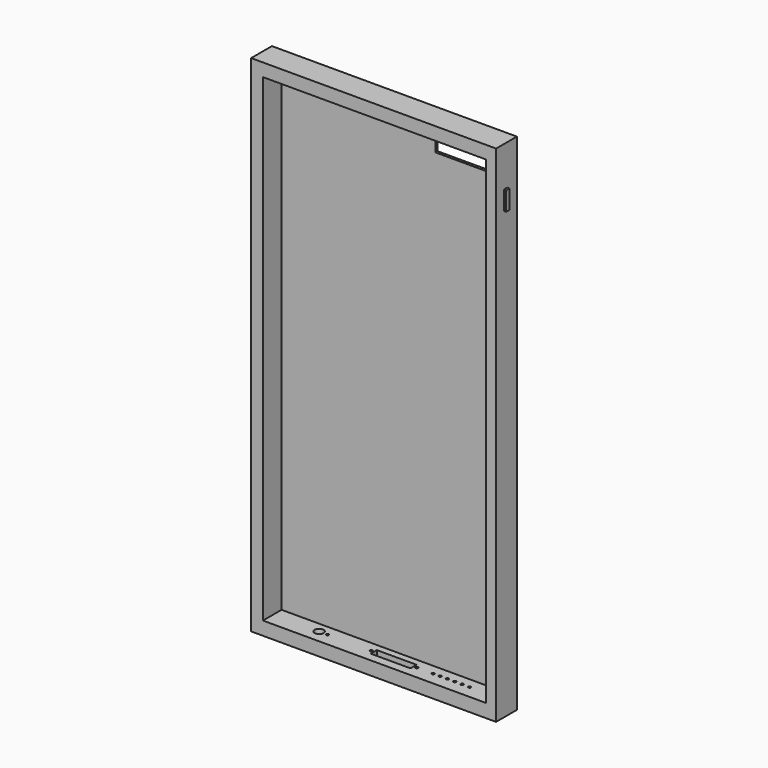
from build123d import *

# Parameters (mm, degrees)
F0_W          = 67.056
F0_H          = 138.176
F1_DEPTH      = 7.112
F2_W          = 1.1457276996
F2_H          = 5.1557719707
F3_DEPTH      = 0.6604
F4_W          = 1.0838428756
F4_H          = 4.3208114803
F5_DEPTH      = 0.7874
F6_W          = 0.8028652519
F6_H          = 3.1311772764
F6_H_2        = 3.1713172793
F7_DEPTH      = 0.4826
F8_W          = 61.0314477235
F8_H          = 130.9745721519
F9_DEPTH      = 6.3754
F10_W         = 17.1431452036
F10_H         = 5.4619573057
F11_DEPTH     = 25.4
F12_TEXT_SIZE = 1.3546895893
F13_DEPTH     = 0.127
F14_TEXT_SIZE = 2.2497099878
F15_DEPTH     = 0.127
F16_R         = 1.2281483903
F17_DEPTH     = 25.4
F18_R         = 0.3683
F19_DEPTH     = 25.4
F20_W         = 10.8844151255
F20_H         = 2.1005012095
F21_DEPTH     = 25.4
F22_DEPTH     = 25.4


# Not quite as in the source:
# - Text() gives the source's letters only with a copy of the font that has no kerning and outlines rounded to 1/6400 em; it was checked with that copy


with BuildPart() as f1:
    # F0 (on Front) → F1 (new body)
    with BuildSketch(Plane.XZ):
        with Locations((-11.8578484981, -4.7733456488)):
            Rectangle(F0_W, F0_H)
    extrude(amount=F1_DEPTH)

    # F2 (on face) → F3 (join)
    with BuildSketch(Plane.YZ.offset(21.6701515019)):
        with Locations((-3.914569621, 50.7939383388)):
            Rectangle(F2_W, F2_H)
    extrude(amount=F3_DEPTH)

    # F4 (on face) → F5 (cut)
    with BuildSketch(Plane(origin=(-45.3858484981, 0, 0), x_dir=(0, -1, 0), z_dir=(-1, 0, 0))):
        with Locations((3.0140785622, 55.3201716393)):
            Rectangle(F4_W, F4_H)
    extrude(amount=-F5_DEPTH, mode=Mode.SUBTRACT)

    # F6 (on face) → F7 (join)
    with BuildSketch(Plane(origin=(-45.3858484981, 0, 0), x_dir=(0, -1, 0), z_dir=(-1, 0, 0))):
        with Locations((3.031330416, 46.9237361103)):
            Rectangle(F6_W, F6_H)
        with Locations((3.031330416, 42.3674732447)):
            Rectangle(F6_W, F6_H_2)
    extrude(amount=F7_DEPTH)

    # F8 (on face) → F9 (cut)
    with BuildSketch(Plane.XZ.offset(7.112)):
        with Locations((-11.6356713697, -4.7019440681)):
            Rectangle(F8_W, F8_H)
    extrude(amount=-F9_DEPTH, mode=Mode.SUBTRACT)

    # F10 (on face) → F11 (cut)
    with BuildSketch(Plane.XZ.offset(0.7366)):
        with Locations((8.5715726018, 56.4674008638)):
            Rectangle(F10_W, F10_H)
    extrude(amount=-F11_DEPTH, mode=Mode.SUBTRACT)

    # F12 (on face) → F13 (join)
    with BuildSketch(Plane(origin=(-45.8684484981, 0, 0), x_dir=(0, -1, 0), z_dir=(-1, 0, 0))):
        with Locations((2.62989779, 46.3512829981)):
            Text('+', F12_TEXT_SIZE, font='Open Sans', font_style=FontStyle.BOLD, text_align=(TextAlign.LEFT, TextAlign.BOTTOM))
    extrude(amount=F13_DEPTH)

    # F14 (on face) → F15 (join)
    with BuildSketch(Plane(origin=(-45.8684484981, 0, 0), x_dir=(0, -1, 0), z_dir=(-1, 0, 0))):
        with Locations((2.62989779, 41.7270419659)):
            Text('-', F14_TEXT_SIZE, font='Open Sans', font_style=FontStyle.BOLD, text_align=(TextAlign.LEFT, TextAlign.BOTTOM))
    extrude(amount=F15_DEPTH)

    # F16 (on face) → F17 (cut)
    with BuildSketch(Plane(origin=(0, 0, -73.8613456488), x_dir=(1, 0, 0), z_dir=(0, 0, -1))):
        with Locations((-29.6269077808, 3.5309551749)):
            Circle(F16_R)
    extrude(amount=-F17_DEPTH, mode=Mode.SUBTRACT)

    # F18 (on face) → F19 (cut)
    with BuildSketch(Plane(origin=(0, 0, -73.8613456488), x_dir=(1, 0, 0), z_dir=(0, 0, -1))):
        with Locations((-27.3215491325, 3.5574366339)):
            Circle(F18_R)
        with Locations((-15.3702935204, 3.5574366339)):
            Circle(F18_R)
        with Locations((-2.9175728559, 3.5574366339)):
            Circle(F18_R)
        with Locations((1.5904586762, 3.5574366339)):
            Circle(F18_R)
        with Locations((3.496132791, 3.5574366339)):
            Circle(F18_R)
        with Locations((5.5014388636, 3.5574366339)):
            Circle(F18_R)
        with Locations((7.5141410343, 3.5574366339)):
            Circle(F18_R)
        with Locations((9.5153255388, 3.5574366339)):
            Circle(F18_R)
        with Locations((11.5590859205, 3.5574366339)):
            Circle(F18_R)
    extrude(amount=-F19_DEPTH, mode=Mode.SUBTRACT)

    # F20 (on face) → F21 (cut)
    with BuildSketch(Plane(origin=(0, 0, -73.8613456488), x_dir=(1, 0, 0), z_dir=(0, 0, -1))):
        with Locations((-9.165823576, 3.6281384528)):
            Rectangle(F20_W, F20_H)
    extrude(amount=-F21_DEPTH, mode=Mode.SUBTRACT)

    # F18 (on face) → F22 (cut)
    with BuildSketch(Plane(origin=(0, 0, -73.8613456488), x_dir=(1, 0, 0), z_dir=(0, 0, -1))):
        with Locations((-27.3215491325, 3.5574366339)):
            Circle(F18_R)
        with Locations((-15.3702935204, 3.5574366339)):
            Circle(F18_R)
        with Locations((-2.9175728559, 3.5574366339)):
            Circle(F18_R)
        with Locations((1.5904586762, 3.5574366339)):
            Circle(F18_R)
        with Locations((3.496132791, 3.5574366339)):
            Circle(F18_R)
        with Locations((5.5014388636, 3.5574366339)):
            Circle(F18_R)
        with Locations((7.5141410343, 3.5574366339)):
            Circle(F18_R)
        with Locations((9.5153255388, 3.5574366339)):
            Circle(F18_R)
        with Locations((11.5590859205, 3.5574366339)):
            Circle(F18_R)
    extrude(amount=-F22_DEPTH, mode=Mode.SUBTRACT)


solid = f1.part
